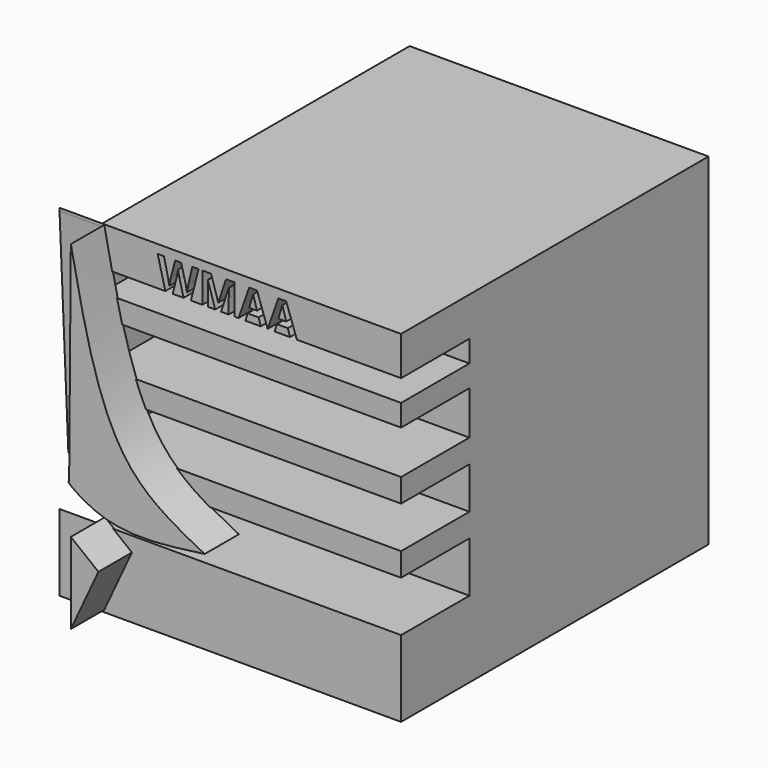
from build123d import *

# Parameters (mm, degrees)
F0_W          = 177.8
F0_H          = 203.2
F1_DEPTH      = 177.8
F2_W          = 177.8
F2_H          = 12.9417330027
F2_H_2        = 13.9372590929
F2_H_3        = 13.9372609556
F2_H_4        = 45.4565609217
F3_DEPTH      = 50.8
F4_W          = 177.8
F4_H          = 23.1797930956
F5_DEPTH      = 50.8
F8_DEPTH      = 25.4
F10_DEPTH     = 25.4
F12_DEPTH     = 25.4
F13_TEXT_SIZE = 25.1796200044
F14_DEPTH     = 25.4


# Not quite as in the source:
# - Text() gives the source's letters only with a copy of the font that has no kerning and outlines rounded to 1/6400 em; it was checked with that copy


with BuildPart() as f1:
    # F0 (on Front) → F1 (new body)
    with BuildSketch(Plane.XZ):
        Rectangle(F0_W, F0_H)
    extrude(amount=F1_DEPTH)

    # F2 (on face) → F3 (join)
    with BuildSketch(Plane.XZ.offset(177.8)):
        with Locations((0, 59.0075962245)):
            Rectangle(F2_W, F2_H)
        with Locations((0, 19.6846164763)):
            Rectangle(F2_W, F2_H_2)
        with Locations((0, -19.1406048834)):
            Rectangle(F2_W, F2_H_3)
        with Locations((0, -78.8717195392)):
            Rectangle(F2_W, F2_H_4)
    extrude(amount=F3_DEPTH)

    # F4 (on face) → F5 (join)
    with BuildSketch(Plane.XZ.offset(177.8)):
        with Locations((0, 90.0101034522)):
            Rectangle(F4_W, F4_H)
    extrude(amount=F5_DEPTH)

    # F7 (on offset) → F8 (join)
    with BuildSketch(Plane.XZ.offset(228.092)):
        with BuildLine():
            add(Edge.make_bspline(
                [(-87.6636505127, 101.3171374798), (-79.8609207381, 62.3668793883), (-66.2530058957, -5.5621416736), (-25.4351900159, -26.2453658301), (-8.0221639946, -35.0689031184)],
                knots=[0, 0, 0, 0, 0.5733964288, 1, 1, 1, 1], degree=3))
            Line((-87.6636505127, 101.3171374798), (-88.6591672897, -23.6204396933))
            add(Edge.make_bspline(
                [(-8.0221639946, -35.0689031184), (-29.7985995613, -38.0933031204), (-64.9126501043, -42.9700853746), (-90.7202378057, -23.2092649558), (-88.8935735145, -23.5736766558), (-88.6591672897, -23.6204396933)],
                knots=[0, 0, 0, 0, 0.5873210988, 0.9470430863, 1, 1, 1, 1], degree=3))
        make_face()
        Polygon((-71.2375938892, -64.9344623089), (-87.6636505127, -51.9927181304), (-87.6636505127, -100.2753674984), align=None)
    extrude(amount=F8_DEPTH)

    # F9 (on face) → F10 (join)
    with BuildSketch(Plane(origin=(-88.9, 0, 0), x_dir=(0, -1, 0), z_dir=(-1, 0, 0))):
        with BuildLine():
            Line((228.5930862524, 99.8963755563), (228.6, 101.6))
            add(Edge.make_bspline(
                [(228.6, 101.6), (208.9651080755, 64.3968583821), (174.4752665061, -0.9526462253), (139.9123926473, -35.4180834028), (125.0259876251, -50.2625219524)],
                knots=[0, 0, 0, 0, 0.5692949295, 1, 1, 1, 1], degree=3))
            add(Edge.make_bspline(
                [(125.0259876251, -50.2625219524), (146.1530221264, -49.4090424469), (182.8279844444, -47.9274654324), (210.5284945222, -35.1681657863), (222.012264945, -29.4328552024)],
                knots=[0, 0, 0, 0, 0.5327490824, 0.9248128279, 0.9248128279, 0.9248128279, 0.9248128279], degree=3))
            Line((222.012264945, -29.4328552024), (228.5930862524, 99.8963755563))
        make_face()
        Polygon((228.6, 100.0322476029), (228.6, 101.6), (228.5930862524, 99.8963755563), align=None)
        Polygon((228.6, -101.6), (228.6, -56.1434390783), (206.9639265537, -81.2518745661), align=None)
    extrude(amount=F10_DEPTH)

    # F11 (on face) → F12 (cut)
    with BuildSketch(Plane(origin=(-88.9, 0, 0), x_dir=(0, -1, 0), z_dir=(-1, 0, 0))):
        with BuildLine():
            Line((57.8411146998, -13.8518605381), (57.8411146998, 54.7872111201))
            add(Edge.make_bspline(
                [(57.8411146998, 54.7872111201), (49.4595009019, 33.2369959106), (36.1090186364, -1.0888240219), (21.5117093609, -10.3900648326), (16.0787887871, -13.8518605381)],
                knots=[0, 0, 0, 0, 0.6278135599, 1, 1, 1, 1], degree=3))
            add(Edge.make_bspline(
                [(16.0787887871, -13.8518605381), (29.9995640914, -13.8518605381), (43.9203393956, -13.8518605381), (57.8411146998, -13.8518605381)],
                knots=[0, 0, 0, 0, 41.7623259127, 41.7623259127, 41.7623259127, 41.7623259127], degree=3))
        make_face()
        with BuildLine():
            add(Edge.make_bspline(
                [(64.4569322467, 54.7872111201), (69.7909125752, 36.5054423619), (79.362209591, 3.700627199), (99.984125652, -9.6121171726), (109.1136708856, -15.5058130622)],
                knots=[0, 0, 0, 0, 0.5572891866, 1, 1, 1, 1], degree=3))
            Line((64.4569322467, 54.7872111201), (64.4569322467, -13.8518605381))
            add(Edge.make_bspline(
                [(109.1136708856, -15.5058130622), (94.2280913393, -14.9544955542), (79.342511793, -14.4031780461), (64.4569322467, -13.8518605381)],
                knots=[0, 0, 0, 0, 44.6873568788, 44.6873568788, 44.6873568788, 44.6873568788], degree=3))
        make_face()
        Polygon((72.7266967297, -33.6993038654), (59.4950690866, -20.4676743597), (50.3983236849, -33.6993038654), (64.4569322467, -52.7197681367), align=None)
    extrude(amount=-F12_DEPTH, mode=Mode.SUBTRACT)

    # F13 (on face) → F14 (cut)
    with BuildSketch(Plane.XZ.offset(228.6)):
        with Locations((-55.9095367789, 78.4202069044)):
            Text('WMAA', F13_TEXT_SIZE, font='Open Sans', font_style=FontStyle.BOLD, text_align=(TextAlign.LEFT, TextAlign.BOTTOM))
    extrude(amount=-F14_DEPTH, mode=Mode.SUBTRACT)


solid = f1.part
